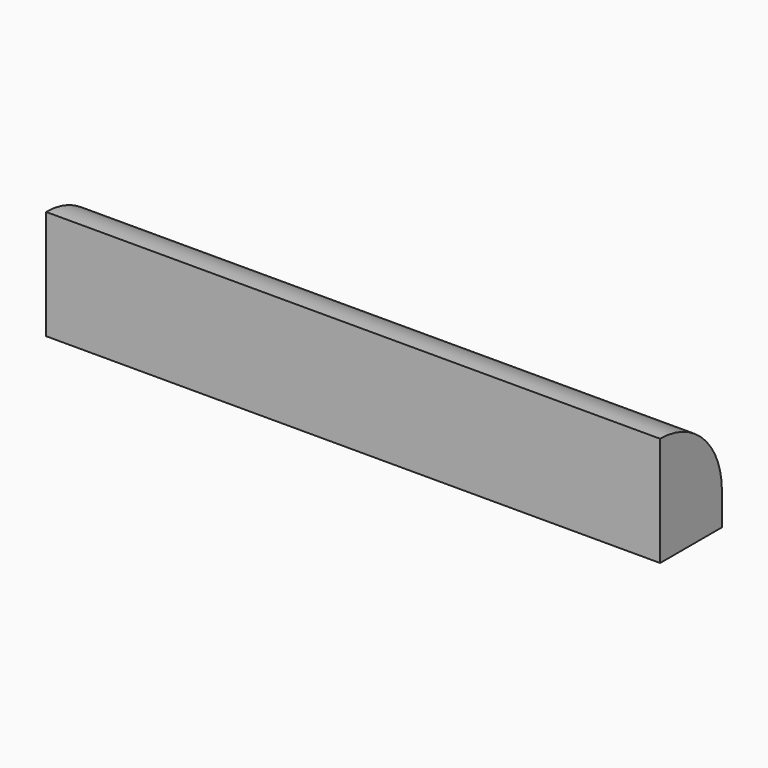
from build123d import *

# Parameters (mm, degrees)
F0_W     = 47.7
F0_H     = 6
F1_DEPTH = 8.5
F2_R     = 5.99999


# Not quite as in the source:
# - a fillet or chamfer is up to 0.001 mm smaller than in the source, because OpenCascade refuses the exact size


with BuildPart() as f1:
    # F0 (on Top) → F1 (new body)
    with BuildSketch(Plane.XY):
        Rectangle(F0_W, F0_H)
    extrude(amount=F1_DEPTH)

    # F2 (radius 6 in the source; OpenCascade refuses exactly that, so slightly less here)
    f2_edges = [f1.edges().sort_by_distance(p)[0] for p in [
        (0, 3, 8.5),
    ]]
    fillet(f2_edges, radius=F2_R)


solid = f1.part
